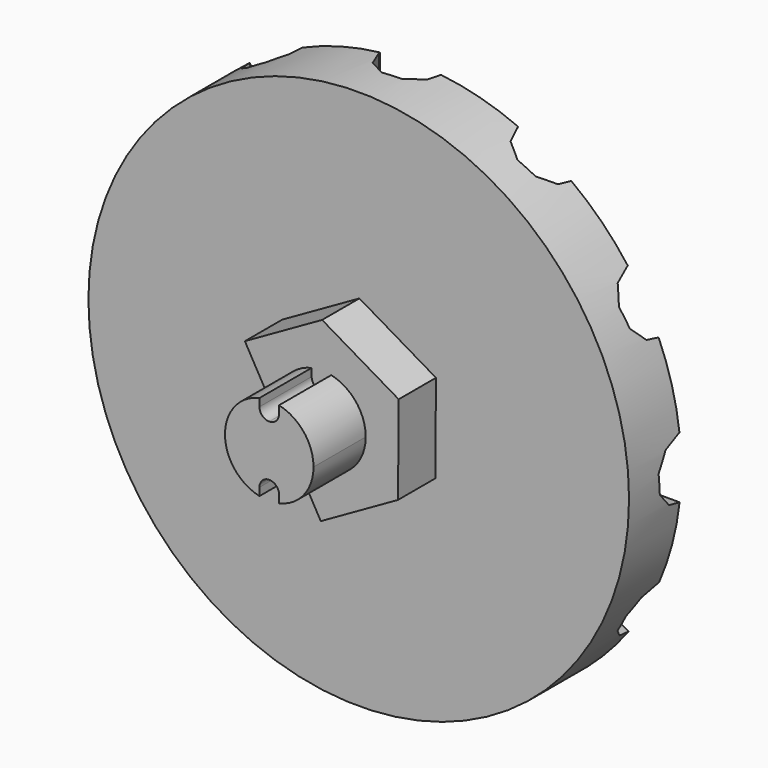
from build123d import *

# Parameters (mm, degrees)
F0_R            = 29
F1_DEPTH        = 7
F3_DEPTH        = 12
F6_DEPTH        = 11
F6_COPIES_COUNT = 12
F9_DEPTH        = 5
F11_DEPTH       = 3.2
F13_DEPTH       = 15


# Not quite as in the source:
# - a pattern or mirror of a feature is missing from the dataset's text; its kind, count and spacing are read off the source's solid


with BuildPart() as f1:
    # F0 (on Front) → F1 (new body)
    with BuildSketch(Plane.XZ):
        Circle(F0_R)
    extrude(amount=F1_DEPTH)

    # F2 (on face) → F3 (join)
    with BuildSketch(Plane.XZ.offset(7)):
        with BuildLine():
            Line((0, -2.75), (0, 2.75))
            ThreePointArc((0, 2.75), (-0.7424621202, 3.0575378798), (-1.05, 3.8))
            Line((-1.05, 3.8), (-1.05, 4.6324939288))
            ThreePointArc((-1.05, 4.6324939288), (-4.75, 0), (-1.05, -4.6324939288))
            Line((-1.05, -4.6324939288), (-1.05, -3.8))
            ThreePointArc((-1.05, -3.8), (-0.7424621202, -3.0575378798), (0, -2.75))
        make_face()
        with BuildLine():
            ThreePointArc((1.05, -4.6324939288), (3.711468712, -2.9643717716), (4.75, 0))
            ThreePointArc((4.75, 0), (3.711468712, 2.9643717716), (1.05, 4.6324939288))
            Line((1.05, 4.6324939288), (1.05, 3.8))
            ThreePointArc((1.05, 3.8), (0.7424621202, 3.0575378798), (0, 2.75))
            Line((0, 2.75), (0, -2.75))
            ThreePointArc((0, -2.75), (0.7424621202, -3.0575378798), (1.05, -3.8))
            Line((1.05, -3.8), (1.05, -4.6324939288))
        make_face()
    extrude(amount=F3_DEPTH)

    # F5 (on offset) → F6 (cut)
    with BuildSketch(Plane.YZ.offset(29)):
        Polygon((-2.8396848584, -1.3322586236), (-1.4665255865, -2.8938910614), (0.5622881169, -3.3501554734), (2.4718183739, -2.5267743623), (3.5326895289, -0.7382513266), (3.3396848584, 1.3322586236), (1.9665255865, 2.8938910614), (-0.0622881169, 3.3501554734), (-1.9718183739, 2.5267743623), (-3.0326895289, 0.7382513266), align=None)
    f6 = extrude(amount=-F6_DEPTH, mode=Mode.SUBTRACT)

    # F6_copies: F6 ×12 about axis
    f6_copies_axis = Axis((0, 0, 0), (0, 1, 0))
    for i in range(1, F6_COPIES_COUNT):
        add(f6.rotate(f6_copies_axis, i * 360 / F6_COPIES_COUNT), mode=Mode.SUBTRACT)

    # F8 (on face) → F9 (join)
    with BuildSketch(Plane.XZ.offset(7)):
        Polygon((8.2854374709, 4.7012260014), (0.0713375892, 9.5260123319), (-8.2140998816, 4.8247863305), (-0.0713375892, -9.5260123319), (8.2140998816, -4.8247863305), align=None)
        with BuildLine():
            ThreePointArc((-1.05, -4.6324939288), (-4.75, 0), (-1.05, 4.6324939288))
            Line((-1.05, 4.6324939288), (-1.05, 3.8))
            ThreePointArc((-1.05, 3.8), (0, 2.75), (1.05, 3.8))
            Line((1.05, 3.8), (1.05, 4.6324939288))
            ThreePointArc((1.05, 4.6324939288), (4.75, 0), (1.05, -4.6324939288))
            Line((1.05, -4.6324939288), (1.05, -3.8))
            ThreePointArc((1.05, -3.8), (0, -2.75), (-1.05, -3.8))
            Line((-1.05, -3.8), (-1.05, -4.6324939288))
        make_face(mode=Mode.SUBTRACT)
        with BuildLine():
            Line((-1.05, 3.8), (-1.05, 4.6324939288))
            ThreePointArc((-1.05, 4.6324939288), (-4.75, 0), (-1.05, -4.6324939288))
            Line((-1.05, -4.6324939288), (-1.05, -3.8))
            ThreePointArc((-1.05, -3.8), (0, -2.75), (1.05, -3.8))
            Line((1.05, -3.8), (1.05, -4.6324939288))
            ThreePointArc((1.05, -4.6324939288), (4.75, 0), (1.05, 4.6324939288))
            Line((1.05, 4.6324939288), (1.05, 3.8))
            ThreePointArc((1.05, 3.8), (0, 2.75), (-1.05, 3.8))
        make_face()
    extrude(amount=F9_DEPTH)

    # F10 (on face) → F11 (cut)
    with BuildSketch(Plane.XZ.offset(7)):
        Polygon((4.92104771, 2.7922433221), (0.0423702045, 5.6578739911), (-4.8786775054, 2.865630669), (-4.92104771, -2.7922433221), (-0.0423702045, -5.6578739911), (4.8786775054, -2.865630669), align=None)
        Polygon((-4.92104771, -2.7922433221), (-4.8786775054, 2.865630669), (-9.9290630252, 0), (-5.0927557243, -8.5235046601), (-0.0423702045, -5.6578739911), align=None)
    extrude(amount=F11_DEPTH, mode=Mode.SUBTRACT)

    # F12 (on face) → F13 (cut)
    with BuildSketch(Plane(origin=(0, 0, 0), x_dir=(-1, 0, 0), z_dir=(0, 1, 0))):
        Polygon((2.9053820181, 0.8348685994), (1.8597799775, 2.3831635875), (0.103805197, 3.0211710859), (-1.6918196405, 2.5051939154), (-2.8412268781, 1.0323178175), (-2.9053820181, -0.8348685994), (-1.8597799775, -2.3831635875), (-0.103805197, -3.0211710859), (1.6918196405, -2.5051939154), (2.8412268781, -1.0323178175), align=None)
    extrude(amount=-F13_DEPTH, mode=Mode.SUBTRACT)


solid = f1.part
